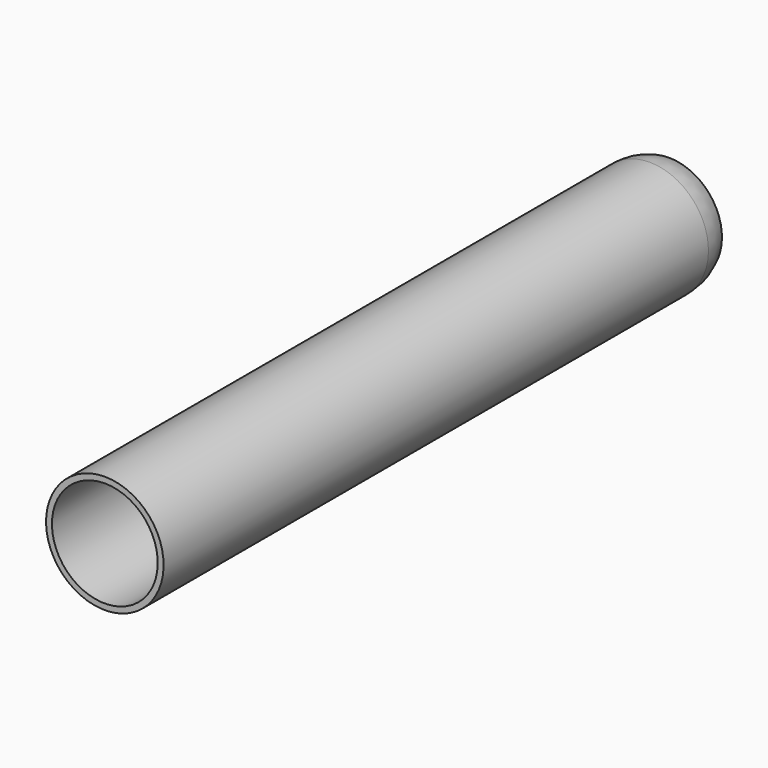
from build123d import *

# Parameters (mm, degrees)
F0_W = 304.8
F0_H = 25.4
F2_T = -2.54


# Not quite as in the source:
# - a fillet or chamfer that OpenCascade refuses, or shapes differently, is made with other operations: its cross-section is extruded or revolved along the edge and cut away or added


with BuildPart() as f1:
    # F0 (on Right) → F1 (revolve)
    with BuildSketch(Plane.YZ):
        Rectangle(F0_W, F0_H)
    revolve(axis=Axis((0, 0, -12.7), (0, -1, 0)))

    # F2
    f2_openings = [f1.faces().sort_by_distance(p)[0] for p in [
        (0, 152.4, -12.7),
        (0, -152.4, -12.7),
    ]]
    offset(amount=F2_T, openings=f2_openings)

    # F3: fillet of radius 22.86 on 1 edges, made by hand

    # F3_s1 → F3_t2 (revolve, cut)
    with BuildSketch(Plane.YZ):
        with BuildLine():
            ThreePointArc((141.9273117109, 12.7), (147.3154653836, 12.0559267194), (152.4, 10.16))
            Line((152.4, 10.16), (152.4, 12.7))
            Line((152.4, 12.7), (141.9273117109, 12.7))
        make_face()
    revolve(axis=Axis((0, 152.4, -12.7), (0, -1, 0)), mode=Mode.SUBTRACT)


solid = f1.part
